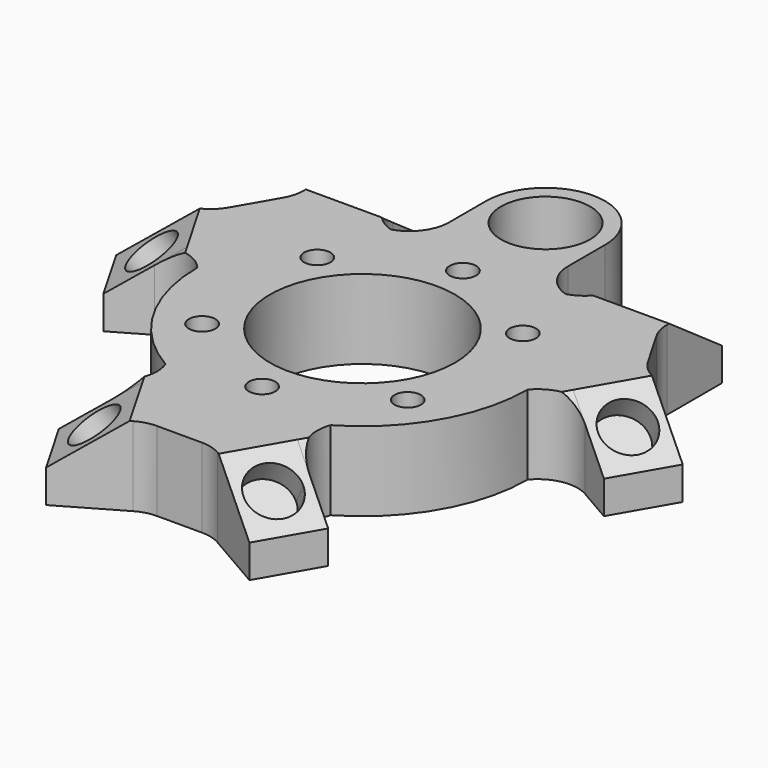
from build123d import *

# Parameters (mm, degrees)
F0_W          = 10
F0_H          = 12
F0_R          = 14
F1_DEPTH      = 12
F2_SIZE2      = 10
F2_SIZE       = 7
F2_2_SIZE2    = 10
F2_2_SIZE     = 7
F2_3_SIZE2    = 10
F2_3_SIZE     = 7
F2_4_SIZE2    = 10
F2_4_SIZE     = 7
F2_5_SIZE2    = 10
F2_5_SIZE     = 7
F2_6_SIZE2    = 10
F2_6_SIZE     = 7
F3_R          = 3.8
F4_DEPTH      = 4
F5_R          = 3.8
F6_DEPTH      = 4
F8_DEPTH      = 4
F9_R          = 2
F10_DEPTH     = 25
F11_T1_DEPTH  = 12
F11_T6_DEPTH  = 12
F11_T11_DEPTH = 12
F11_T16_DEPTH = 12
F11_T21_DEPTH = 12
F11_T26_DEPTH = 12
F11_T31_DEPTH = 12


# Not quite as in the source:
# - a fillet or chamfer that OpenCascade refuses, or shapes differently, is made with other operations: its cross-section is extruded or revolved along the edge and cut away or added


with BuildPart() as f1:
    # F0 (on Top) → F1 (new body)
    with BuildSketch(Plane.XY):
        with Locations((-22.5, 27.6506350946)):
            Rectangle(F0_W, F0_H)
        with BuildLine():
            Line((-9, 34.6506350946), (-9, 21.6506350946))
            Line((-9, 21.6506350946), (0, 21.6506350946))
            Line((0, 21.6506350946), (9, 21.6506350946))
            Line((9, 21.6506350946), (9, 34.6506350946))
            ThreePointArc((9, 34.6506350946), (0, 43.6506350946), (-9, 34.6506350946))
        make_face()
        with BuildLine():
            ThreePointArc((6.75, 34.6506350946), (4.772970773, 29.8776643216), (0, 27.9006350946))
            ThreePointArc((0, 27.9006350946), (-4.772970773, 39.4236058676), (6.75, 34.6506350946))
        make_face(mode=Mode.SUBTRACT)
        with Locations((22.5, 27.6506350946)):
            Rectangle(F0_W, F0_H)
        Polygon((-17.5, 21.6506350946), (-27.5, 21.6506350946), (-32.5, 12.9903810568), (-27.5, 4.3301270189), (-25, 0), (-12.5, -21.6506350946), (-10, -25.9807621135), (-5, -34.6410161514), (5, -34.6410161514), (10, -25.9807621135), (12.5, -21.6506350946), (25, 0), (27.5, 4.3301270189), (32.5, 12.9903810568), (27.5, 21.6506350946), (17.5, 21.6506350946), (9, 21.6506350946), (0, 21.6506350946), (-9, 21.6506350946), align=None)
        Circle(F0_R, mode=Mode.SUBTRACT)
        Polygon((42.8923048454, 6.9903810568), (32.5, 12.9903810568), (27.5, 4.3301270189), (37.8923048454, -1.6698729811), align=None)
        Polygon((10, -25.9807621135), (5, -34.6410161514), (15.3923048454, -40.6410161514), (20.3923048454, -31.9807621135), align=None)
        Polygon((-27.5, 4.3301270189), (-32.5, 12.9903810568), (-42.8923048454, 6.9903810568), (-37.8923048454, -1.6698729811), align=None)
        with BuildLine():
            Line((-12.5, -21.6506350946), (-25, 0))
            ThreePointArc((-25, 0), (-21.6506350946, -12.5), (-12.5, -21.6506350946))
        make_face()
        with BuildLine():
            Line((25, 0), (12.5, -21.6506350946))
            ThreePointArc((12.5, -21.6506350946), (21.6506350946, -12.5), (25, 0))
        make_face()
        Polygon((-5, -34.6410161514), (-10, -25.9807621135), (-20.3923048454, -31.9807621135), (-15.3923048454, -40.6410161514), align=None)
    extrude(amount=F1_DEPTH)

    # F2
    f2_edges = [f1.edges().sort_by_distance(p)[0] for p in [
        (-17.892305, -36.310889, 12),
    ]]
    f2_side = f1.faces().sort_by_distance((-17.892305, -36.310889, 6))[0]
    chamfer(f2_edges, length=F2_SIZE, length2=F2_SIZE2, reference=f2_side)

    # F2#2
    f2_2_edges = [f1.edges().sort_by_distance(p)[0] for p in [
        (-40.392305, 2.660254, 12),
    ]]
    f2_2_side = f1.faces().sort_by_distance((-40.392305, 2.660254, 6))[0]
    chamfer(f2_2_edges, length=F2_2_SIZE, length2=F2_2_SIZE2, reference=f2_2_side)

    # F2#3
    f2_3_edges = [f1.edges().sort_by_distance(p)[0] for p in [
        (-22.5, 33.650635, 12),
    ]]
    f2_3_side = f1.faces().sort_by_distance((-22.5, 33.650635, 6))[0]
    chamfer(f2_3_edges, length=F2_3_SIZE, length2=F2_3_SIZE2, reference=f2_3_side)

    # F2#4
    f2_4_edges = [f1.edges().sort_by_distance(p)[0] for p in [
        (22.5, 33.650635, 12),
    ]]
    f2_4_side = f1.faces().sort_by_distance((22.5, 33.650635, 6))[0]
    chamfer(f2_4_edges, length=F2_4_SIZE, length2=F2_4_SIZE2, reference=f2_4_side)

    # F2#5
    f2_5_edges = [f1.edges().sort_by_distance(p)[0] for p in [
        (40.392305, 2.660254, 12),
    ]]
    f2_5_side = f1.faces().sort_by_distance((40.392305, 2.660254, 6))[0]
    chamfer(f2_5_edges, length=F2_5_SIZE, length2=F2_5_SIZE2, reference=f2_5_side)

    # F2#6
    f2_6_edges = [f1.edges().sort_by_distance(p)[0] for p in [
        (17.892305, -36.310889, 12),
    ]]
    f2_6_side = f1.faces().sort_by_distance((17.892305, -36.310889, 6))[0]
    chamfer(f2_6_edges, length=F2_6_SIZE, length2=F2_6_SIZE2, reference=f2_6_side)

    # F3 (on face) → F4 (cut)
    with BuildSketch(Plane(origin=(-11.6179988507, -6.7076547639, 19.1647278968), x_dir=(0.8679606585, -0.1640629087, 0.4687511678), z_dir=(-0.4966329583, -0.2867311722, 0.8192319205))):
        with Locations((-28.1627729742, 7.6785275048)):
            Circle(F3_R)
        with Locations((-2.2399390534, -29.1047116336)):
            Circle(F3_R)
    extrude(amount=-F4_DEPTH, mode=Mode.SUBTRACT)

    # F5 (on face) → F6 (cut)
    with BuildSketch(Plane(origin=(0, 13.4153095278, 19.1647278968), x_dir=(1, 0, 0), z_dir=(0, 0.5734623444, 0.8192319205))):
        with BuildLine():
            ThreePointArc((18.7, 18.5970848856), (22.5, 14.7970848856), (26.3, 18.5970848856))
            Line((26.3, 18.5970848856), (22.5, 18.5970848856))
            Line((22.5, 18.5970848856), (18.7, 18.5970848856))
        make_face()
        with BuildLine():
            Line((22.5, 18.5970848856), (26.3, 18.5970848856))
            ThreePointArc((26.3, 18.5970848856), (22.5, 22.3970848856), (18.7, 18.5970848856))
            Line((18.7, 18.5970848856), (22.5, 18.5970848856))
        make_face()
        with Locations((-22.5, 18.5970848856)):
            Circle(F5_R)
    extrude(amount=-F6_DEPTH, mode=Mode.SUBTRACT)

    # F7 (on face) → F8 (cut)
    with BuildSketch(Plane(origin=(11.6179988507, -6.7076547639, 19.1647278968), x_dir=(0.8679606585, 0.1640629087, -0.4687511678), z_dir=(0.4966329583, -0.2867311722, 0.8192319205))):
        with BuildLine():
            Line((2.2399390534, -29.1047116336), (0.0508997446, -32.2108518276))
            ThreePointArc((0.0508997446, -32.2108518276), (3.9894605061, -32.4780148644), (6.0399390534, -29.1047116336))
            ThreePointArc((6.0399390534, -29.1047116336), (5.6132422842, -27.355190181), (4.4289783623, -25.9985714397))
            Line((4.4289783623, -25.9985714397), (2.2399390534, -29.1047116336))
        make_face()
        with BuildLine():
            ThreePointArc((4.4289783623, -25.9985714397), (-0.8662011405, -26.9156723248), (0.0508997446, -32.2108518276))
            Line((0.0508997446, -32.2108518276), (2.2399390534, -29.1047116336))
            Line((2.2399390534, -29.1047116336), (4.4289783623, -25.9985714397))
        make_face()
        with BuildLine():
            ThreePointArc((31.9627729742, 7.6785275048), (26.4132515216, 11.0518307356), (25.9737336654, 4.5723873109))
            ThreePointArc((25.9737336654, 4.5723873109), (29.9122944269, 4.305224274), (31.9627729742, 7.6785275048))
        make_face()
    extrude(amount=-F8_DEPTH, mode=Mode.SUBTRACT)

    # F9 (on face) → F10 (cut)
    with BuildSketch(Plane.XY.offset(12)):
        with Locations((-15.5638888415, 10.8979522907)):
            Circle(F9_R)
        with Locations((0, 19)):
            Circle(F9_R)
        with Locations((-15.5638888415, -10.8979522907)):
            Circle(F9_R)
        with Locations((0, -19)):
            Circle(F9_R)
        with Locations((15.5638888415, -10.8979522907)):
            Circle(F9_R)
        with Locations((15.5638888415, 10.8979522907)):
            Circle(F9_R)
    extrude(amount=-F10_DEPTH, mode=Mode.SUBTRACT)

    # F11: fillet of radius 6 on 14 edges, made by hand

    # F11_s2 → F11_t1 (join)
    with BuildSketch(Plane.XY):
        with BuildLine():
            ThreePointArc((6.3923048454, -35.4448637287), (4.945219116, -34.8454611936), (3.3923048454, -34.6410161514))
            Line((3.3923048454, -34.6410161514), (5, -34.6410161514))
            Line((5, -34.6410161514), (6.3923048454, -35.4448637287))
        make_face()
        with BuildLine():
            ThreePointArc((-3.3923048454, -34.6410161514), (-4.945219116, -34.8454611936), (-6.3923048454, -35.4448637287))
            Line((-6.3923048454, -35.4448637287), (-5, -34.6410161514))
            Line((-5, -34.6410161514), (-3.3923048454, -34.6410161514))
        make_face()
        with BuildLine():
            ThreePointArc((28.3038475773, 20.2583302492), (27.7044450423, 21.7054159786), (27.5, 23.2583302492))
            Line((27.5, 23.2583302492), (27.5, 21.6506350946))
            Line((27.5, 21.6506350946), (28.3038475773, 20.2583302492))
        make_face()
        with BuildLine():
            ThreePointArc((33.8923048454, 12.1865334795), (32.6496641583, 13.1400452151), (31.6961524227, 14.3826859022))
            Line((31.6961524227, 14.3826859022), (32.5, 12.9903810568))
            Line((32.5, 12.9903810568), (33.8923048454, 12.1865334795))
        make_face()
        with BuildLine():
            ThreePointArc((-33.8923048454, 12.1865334795), (-32.6496641583, 13.1400452151), (-31.6961524227, 14.3826859022))
            Line((-31.6961524227, 14.3826859022), (-32.5, 12.9903810568))
            Line((-32.5, 12.9903810568), (-33.8923048454, 12.1865334795))
        make_face()
        with BuildLine():
            ThreePointArc((-28.3038475773, 20.2583302492), (-27.7044450423, 21.7054159786), (-27.5, 23.2583302492))
            Line((-27.5, 23.2583302492), (-27.5, 21.6506350946))
            Line((-27.5, 21.6506350946), (-28.3038475773, 20.2583302492))
        make_face()
        with BuildLine():
            ThreePointArc((15, 21.6506350946), (10.7573593129, 23.4079944075), (9, 27.6506350946))
            Line((9, 27.6506350946), (9, 21.6506350946))
            Line((9, 21.6506350946), (15, 21.6506350946))
        make_face()
        with BuildLine():
            ThreePointArc((-9, 27.6506350946), (-10.7573593129, 23.4079944075), (-15, 21.6506350946))
            Line((-15, 21.6506350946), (-9, 21.6506350946))
            Line((-9, 21.6506350946), (-9, 27.6506350946))
        make_face()
    extrude(amount=F11_T1_DEPTH)


with BuildPart() as f11_tool4:
    # F11_s5 → F11_t6 (new body)
    with BuildSketch(Plane.XY):
        with BuildLine():
            ThreePointArc((15.123475383, -28.9388020051), (12.4780855693, -25.7747848759), (12.5, -21.6506350946))
            Line((12.5, -21.6506350946), (10, -25.9807621135))
            Line((10, -25.9807621135), (15.123475383, -28.9388020051))
        make_face()
    extrude(amount=F11_T6_DEPTH)

    split(bisect_by=Plane(origin=(11.6179988507, -6.7076547639, 19.1647278968), x_dir=(-0.5, -0.8660254038, 0), z_dir=(-0.4966329583, 0.2867311722, -0.8192319205)), keep=Keep.TOP)


with BuildPart() as f1_1:
    add(f1.part)

    # F11_t3: union F11_tool4
    add(f11_tool4.part)


with BuildPart() as f11_tool9:
    # F11_s10 → F11_t11 (new body)
    with BuildSketch(Plane.XY):
        with BuildLine():
            ThreePointArc((25, 0), (28.5606612642, 2.0810533444), (32.623475383, 1.3720871274))
            Line((32.623475383, 1.3720871274), (27.5, 4.3301270189))
            Line((27.5, 4.3301270189), (25, 0))
        make_face()
    extrude(amount=F11_T11_DEPTH)

    split(bisect_by=Plane(origin=(11.6179988507, -6.7076547639, 19.1647278968), x_dir=(-0.5, -0.8660254038, 0), z_dir=(-0.4966329583, 0.2867311722, -0.8192319205)), keep=Keep.TOP)


with BuildPart() as f1_2:
    add(f1_1.part)

    # F11_t8: union F11_tool9
    add(f11_tool9.part)


with BuildPart() as f11_tool14:
    # F11_s15 → F11_t16 (new body)
    with BuildSketch(Plane.XY):
        with BuildLine():
            ThreePointArc((-25, 0), (-28.5606612642, 2.0810533444), (-32.623475383, 1.3720871274))
            Line((-32.623475383, 1.3720871274), (-27.5, 4.3301270189))
            Line((-27.5, 4.3301270189), (-25, 0))
        make_face()
    extrude(amount=F11_T16_DEPTH)

    split(bisect_by=Plane(origin=(-11.6179988507, -6.7076547639, 19.1647278968), x_dir=(-0.5, 0.8660254038, 0), z_dir=(0.4966329583, 0.2867311722, -0.8192319205)), keep=Keep.TOP)


with BuildPart() as f1_3:
    add(f1_2.part)

    # F11_t13: union F11_tool14
    add(f11_tool14.part)


with BuildPart() as f11_tool19:
    # F11_s20 → F11_t21 (new body)
    with BuildSketch(Plane.XY):
        with BuildLine():
            ThreePointArc((17.5, 27.6506350946), (15.7426406871, 23.4079944075), (11.5, 21.6506350946))
            Line((11.5, 21.6506350946), (17.5, 21.6506350946))
            Line((17.5, 21.6506350946), (17.5, 27.6506350946))
        make_face()
    extrude(amount=F11_T21_DEPTH)

    split(bisect_by=Plane(origin=(0, 13.4153095278, 19.1647278968), x_dir=(1, 0, 0), z_dir=(0, -0.5734623444, -0.8192319205)), keep=Keep.TOP)


with BuildPart() as f1_4:
    add(f1_3.part)

    # F11_t18: union F11_tool19
    add(f11_tool19.part)


with BuildPart() as f11_tool24:
    # F11_s25 → F11_t26 (new body)
    with BuildSketch(Plane.XY):
        with BuildLine():
            ThreePointArc((-15.123475383, -28.9388020051), (-12.4780855693, -25.7747848759), (-12.5, -21.6506350946))
            Line((-12.5, -21.6506350946), (-10, -25.9807621135))
            Line((-10, -25.9807621135), (-15.123475383, -28.9388020051))
        make_face()
    extrude(amount=F11_T26_DEPTH)

    split(bisect_by=Plane(origin=(-11.6179988507, -6.7076547639, 19.1647278968), x_dir=(-0.5, 0.8660254038, 0), z_dir=(0.4966329583, 0.2867311722, -0.8192319205)), keep=Keep.TOP)


with BuildPart() as f1_5:
    add(f1_4.part)

    # F11_t23: union F11_tool24
    add(f11_tool24.part)


with BuildPart() as f11_tool29:
    # F11_s30 → F11_t31 (new body)
    with BuildSketch(Plane.XY):
        with BuildLine():
            ThreePointArc((-11.5, 21.6506350946), (-15.7426406871, 23.4079944075), (-17.5, 27.6506350946))
            Line((-17.5, 27.6506350946), (-17.5, 21.6506350946))
            Line((-17.5, 21.6506350946), (-11.5, 21.6506350946))
        make_face()
    extrude(amount=F11_T31_DEPTH)

    split(bisect_by=Plane(origin=(0, 13.4153095278, 19.1647278968), x_dir=(1, 0, 0), z_dir=(0, -0.5734623444, -0.8192319205)), keep=Keep.TOP)


with BuildPart() as f1_6:
    add(f1_5.part)

    # F11_t28: union F11_tool29
    add(f11_tool29.part)


solid = f1_6.part
